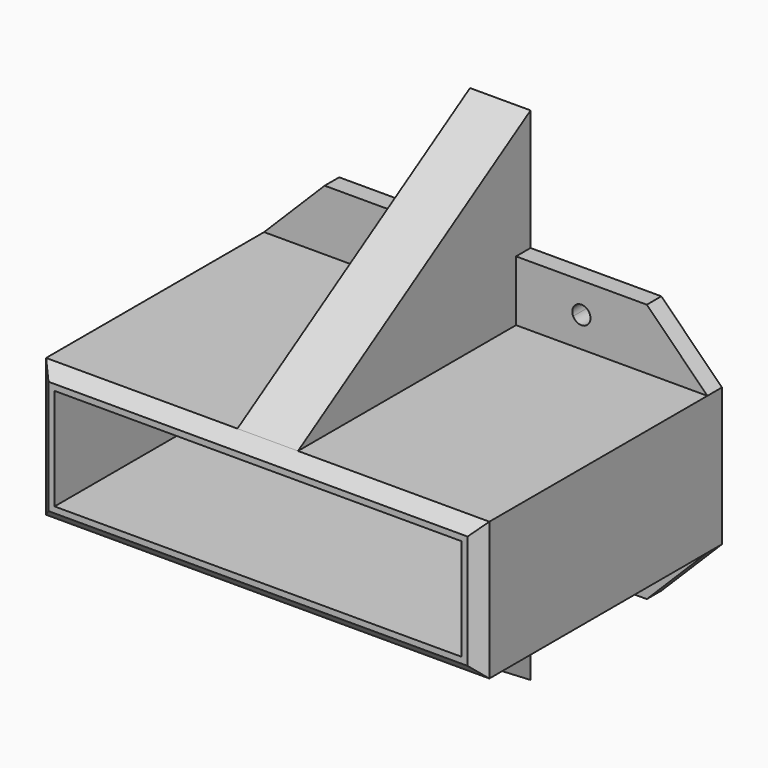
from build123d import *

# Parameters (mm, degrees)
F0_W          = 73.2
F0_H          = 22.8
F0_W_2        = 67.2
F0_H_2        = 16.8
F1_DEPTH      = 50
F2_SIZE       = 2
F3_W          = 9.9999998882
F3_H          = 48
F4_DEPTH      = 30
F6_DEPTH      = 25
F7_W          = 9.9999998882
F7_H          = 48
F8_DEPTH      = 30
F10_DEPTH     = 25
F11_W         = 31.6
F11_H         = 3
F12_W         = 31.6000001118
F12_H         = 3
F13_DEPTH     = 10
F14_T1_DEPTH  = 54.4336597593
F14_T6_DEPTH  = 84.2336597593
F14_T11_DEPTH = 83.0336598711
F14_T16_DEPTH = 83.0336597593
F14_T21_DEPTH = 84.2336597593
F16_DEPTH     = 25
F18_DEPTH     = 25


# Not quite as in the source:
# - a fillet or chamfer that OpenCascade refuses, or shapes differently, is made with other operations: its cross-section is extruded or revolved along the edge and cut away or added


with BuildPart() as f1:
    # F0 (on Front) → F1 (new body)
    with BuildSketch(Plane.XZ):
        Rectangle(F0_W, F0_H)
        Rectangle(F0_W_2, F0_H_2, mode=Mode.SUBTRACT)
    extrude(amount=F1_DEPTH)

    # F2
    f2_edges = [f1.edges().sort_by_distance(p)[0] for p in [
        (-36.6, -50, 0),
        (0, -50, 11.4),
        (36.6, -50, 0),
        (0, -50, -11.4),
    ]]
    chamfer(f2_edges, length=F2_SIZE)

    # F3 (on face) → F4 (join)
    with BuildSketch(Plane(origin=(0, 0, -11.4), x_dir=(1, 0, 0), z_dir=(0, 0, -1))):
        with Locations((5.59e-08, 24)):
            Rectangle(F3_W, F3_H)
    extrude(amount=F4_DEPTH)

    # F5 (on face) → F6 (cut)
    with BuildSketch(Plane(origin=(-4.9999998882, 0, 0), x_dir=(0, -1, 0), z_dir=(-1, 0, 0))):
        Polygon((48, -41.4), (48, -11.4), (0, -41.4), align=None)
    extrude(amount=-F6_DEPTH, mode=Mode.SUBTRACT)

    # F7 (on face) → F8 (join)
    with BuildSketch(Plane.XY.offset(11.4)):
        with Locations((-5.59e-08, -24)):
            Rectangle(F7_W, F7_H)
    extrude(amount=F8_DEPTH)

    # F9 (on face) → F10 (cut)
    with BuildSketch(Plane.YZ.offset(4.9999998882)):
        Polygon((-48, 41.4), (-48, 11.4), (0, 41.4), align=None)
    extrude(amount=-F10_DEPTH, mode=Mode.SUBTRACT)

    # F11 (on face) + F12 (on face) → F13 (join)
    with BuildSketch(Plane.XY.offset(11.4)):
        with Locations((-20.8, -1.5)):
            Rectangle(F11_W, F11_H)
    with BuildSketch(Plane.XY.offset(11.4)):
        with Locations((20.7999999441, -1.5)):
            Rectangle(F12_W, F12_H)
    extrude(amount=F13_DEPTH)

    # F14: chamfer of 10 on 6 edges, made by hand

    # F14_s2 → F14_t1 (cut)
    with BuildSketch(Plane.XZ.offset(-25.7168298797)):
        Polygon((-36.6, 11.4), (-26.6, 21.4), (-36.6, 21.4), align=None)
        Polygon((26.6, 21.4), (36.6, 11.4), (36.6, 21.4), align=None)
    extrude(amount=F14_T1_DEPTH, mode=Mode.SUBTRACT)


with BuildPart() as f14_tool4:
    # F14_s5 → F14_t6 (new body)
    with BuildSketch(Plane.XY.offset(47.1168298797)):
        Polygon((36.6, -10), (26.6, 0), (36.6, 0), align=None)
    extrude(amount=-F14_T6_DEPTH)

    split(bisect_by=Plane(origin=(24, 0, 24), x_dir=(0, 1, 0), z_dir=(0.7071067812, 0, 0.7071067812)), keep=Keep.TOP)


with BuildPart() as f1_1:
    add(f1.part)

    # F14_t3: cut F14_tool4
    add(f14_tool4.part, mode=Mode.SUBTRACT)


with BuildPart() as f14_tool9:
    # F14_s10 → F14_t11 (new body)
    with BuildSketch(Plane.YZ.offset(62.3168298797)):
        Polygon((-10, 21.4), (0, 11.4), (0, 21.4), align=None)
    extrude(amount=-F14_T11_DEPTH)

    split(bisect_by=Plane(origin=(24, 0, 24), x_dir=(0, 1, 0), z_dir=(0.7071067812, 0, 0.7071067812)), keep=Keep.TOP)


with BuildPart() as f1_2:
    add(f1_1.part)

    # F14_t8: cut F14_tool9
    add(f14_tool9.part, mode=Mode.SUBTRACT)


with BuildPart() as f14_tool14:
    # F14_s15 → F14_t16 (new body)
    with BuildSketch(Plane.YZ.offset(20.7168298797)):
        Polygon((-10, 21.4), (0, 11.4), (0, 21.4), align=None)
    extrude(amount=-F14_T16_DEPTH)

    split(bisect_by=Plane(origin=(-24, 0, 24), x_dir=(0, 1, 0), z_dir=(-0.7071067812, 0, 0.7071067812)), keep=Keep.TOP)


with BuildPart() as f1_3:
    add(f1_2.part)

    # F14_t13: cut F14_tool14
    add(f14_tool14.part, mode=Mode.SUBTRACT)


with BuildPart() as f14_tool19:
    # F14_s20 → F14_t21 (new body)
    with BuildSketch(Plane.XY.offset(47.1168298797)):
        Polygon((-36.6, -10), (-26.6, 0), (-36.6, 0), align=None)
    extrude(amount=-F14_T21_DEPTH)

    split(bisect_by=Plane(origin=(-24, 0, 24), x_dir=(0, 1, 0), z_dir=(-0.7071067812, 0, 0.7071067812)), keep=Keep.TOP)


with BuildPart() as f1_4:
    add(f1_3.part)

    # F14_t18: cut F14_tool19
    add(f14_tool19.part, mode=Mode.SUBTRACT)

    # F15 (on face) → F16 (cut)
    with BuildSketch(Plane.XZ.offset(3)):
        with BuildLine():
            Line((-17.1612003607, 15.7698146478), (-15.8, 16.4))
            Line((-15.8, 16.4), (-17.1612003607, 17.0301853522))
            ThreePointArc((-17.1612003607, 17.0301853522), (-17.3, 16.4), (-17.1612003607, 15.7698146478))
        make_face()
        with BuildLine():
            Line((-17.1612003607, 17.0301853522), (-15.8, 16.4))
            Line((-15.8, 16.4), (-14.4387996393, 17.0301853522))
            ThreePointArc((-14.4387996393, 17.0301853522), (-15.8, 17.9), (-17.1612003607, 17.0301853522))
        make_face()
        with BuildLine():
            Line((-15.8, 16.4), (-14.4387996393, 15.7698146478))
            ThreePointArc((-14.4387996393, 15.7698146478), (-14.3351108334, 16.0773551031), (-14.3, 16.4))
            ThreePointArc((-14.3, 16.4), (-14.3351108334, 16.7226448969), (-14.4387996393, 17.0301853522))
            Line((-14.4387996393, 17.0301853522), (-15.8, 16.4))
        make_face()
        with BuildLine():
            ThreePointArc((-17.1612003607, 15.7698146478), (-15.8, 14.9), (-14.4387996393, 15.7698146478))
            Line((-14.4387996393, 15.7698146478), (-15.8, 16.4))
            Line((-15.8, 16.4), (-17.1612003607, 15.7698146478))
        make_face()
    extrude(amount=-F16_DEPTH, mode=Mode.SUBTRACT)

    # F17 (on face) → F18 (cut)
    with BuildSketch(Plane.XZ.offset(3)):
        with BuildLine():
            Line((14.4387995822, 17.0301853495), (15.7999999441, 16.4))
            Line((15.7999999441, 16.4), (17.161200306, 17.0301853495))
            ThreePointArc((17.161200306, 17.0301853495), (15.7999999441, 17.9), (14.4387995822, 17.0301853495))
        make_face()
        with BuildLine():
            Line((17.161200306, 17.0301853495), (15.7999999441, 16.4))
            Line((15.7999999441, 16.4), (17.161200306, 15.7698146505))
            ThreePointArc((17.161200306, 15.7698146505), (17.2648891111, 16.0773551046), (17.2999999441, 16.4))
            ThreePointArc((17.2999999441, 16.4), (17.2648891111, 16.7226448954), (17.161200306, 17.0301853495))
        make_face()
        with BuildLine():
            Line((15.7999999441, 16.4), (14.4387995822, 15.7698146505))
            ThreePointArc((14.4387995822, 15.7698146505), (15.7999999441, 14.9), (17.161200306, 15.7698146505))
            Line((17.161200306, 15.7698146505), (15.7999999441, 16.4))
        make_face()
        with BuildLine():
            ThreePointArc((14.4387995822, 17.0301853495), (14.2999999441, 16.4), (14.4387995822, 15.7698146505))
            Line((14.4387995822, 15.7698146505), (15.7999999441, 16.4))
            Line((15.7999999441, 16.4), (14.4387995822, 17.0301853495))
        make_face()
    extrude(amount=-F18_DEPTH, mode=Mode.SUBTRACT)

    # F19: F1 across plane


with BuildPart() as f1_5:
    add(f1_4.part)
    add(f1_4.part.mirror(Plane.XY))


solid = f1_5.part
